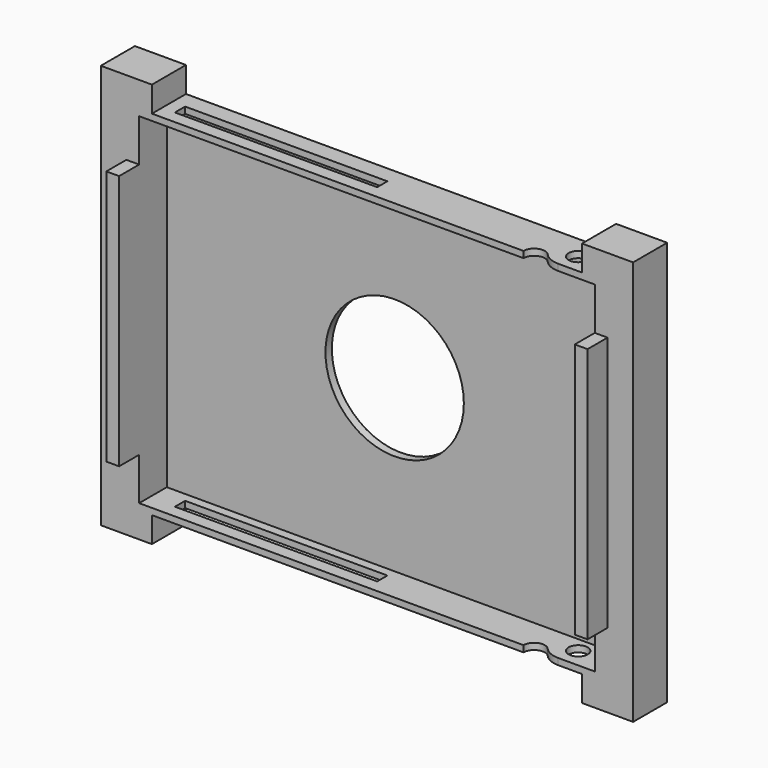
from build123d import *

# Parameters (mm, degrees)
F0_R      = 16.25
F1_DEPTH  = 15.875
F2_W      = 139.2096877098
F2_H      = 115.5483946204
F2_W_2    = 113
F2_H_2    = 80
F3_DEPTH  = 5.875
F4_W      = 107
F4_H      = 80
F5_DEPTH  = 14
F6_W      = 120.5911301091
F6_H      = 13.1527084535
F6_W_2    = 121.3300417974
F6_H_2    = 15.8128053223
F7_DEPTH  = 5.875
F8_R      = 1.5
F8_W      = 89
F8_H      = 3
F9_DEPTH  = 100
F10_W     = 42.4407012761
F10_H     = 10
F11_DEPTH = 1.5
F12_W     = 42.5221920013
F12_H     = 10
F13_DEPTH = 1.5
F14_R     = 2.5
F15_DEPTH = 95.5
F16_R     = 2.25
F17_DEPTH = 200
F18_R     = 5


with BuildPart() as f1:
    # F0 (on Front) → F1 (new body)
    with BuildSketch(Plane.XZ):
        Polygon((-50.5, 47.5), (-62.5, 47.5), (-62.5, -47.5), (-50.5, -47.5), (-50.5, -41.5), (50.5, -41.5), (50.5, -47.5), (62.5, -47.5), (62.5, 47.5), (50.5, 47.5), (50.5, 41.5), (-50.5, 41.5), align=None)
        Circle(F0_R, mode=Mode.SUBTRACT)
    extrude(amount=F1_DEPTH)

    # F2 (on face) → F3 (cut)
    with BuildSketch(Plane.XZ.offset(15.875)):
        Rectangle(F2_W, F2_H)
        Rectangle(F2_W_2, F2_H_2, mode=Mode.SUBTRACT)
    extrude(amount=-F3_DEPTH, mode=Mode.SUBTRACT)

    # F4 (on face) → F5 (cut)
    with BuildSketch(Plane.XZ.offset(15.875)):
        Rectangle(F4_W, F4_H)
    extrude(amount=-F5_DEPTH, mode=Mode.SUBTRACT)

    # F6 (on face) → F7 (cut)
    with BuildSketch(Plane.XZ.offset(15.875)):
        with Locations((0.0607829645, 36.5763542267)):
            Rectangle(F6_W, F6_H)
        with Locations((1.0213727103, -37.9064026611)):
            Rectangle(F6_W_2, F6_H_2)
    extrude(amount=-F7_DEPTH, mode=Mode.SUBTRACT)

    # F8 (on face) → F9 (cut)
    with BuildSketch(Plane.XY.offset(41.5)):
        with Locations((46, -5.5)):
            Circle(F8_R)
        with Locations((-3, -5.5)):
            Rectangle(F8_W, F8_H)
    extrude(amount=-F9_DEPTH, mode=Mode.SUBTRACT)

    # F10 (on face) → F11 (join)
    with BuildSketch(Plane.XY.offset(41.5)):
        with Locations((21.220350638, -5)):
            Rectangle(F10_W, F10_H)
    extrude(amount=-F11_DEPTH)

    # F12 (on face) → F13 (join)
    with BuildSketch(Plane(origin=(0, 0, -41.5), x_dir=(1, 0, 0), z_dir=(0, 0, -1))):
        with Locations((21.2610960007, 5)):
            Rectangle(F12_W, F12_H)
    extrude(amount=-F13_DEPTH)

    # F14 (on face) → F15 (cut)
    with BuildSketch(Plane(origin=(0, 0, -41.5), x_dir=(1, 0, 0), z_dir=(0, 0, -1))):
        with Locations((39.25, 10)):
            Circle(F14_R)
    extrude(amount=-F15_DEPTH, mode=Mode.SUBTRACT)

    # F16 (on face) → F17 (cut)
    with BuildSketch(Plane.XY.offset(41.5)):
        with Locations((46, -5.5)):
            Circle(F16_R)
    extrude(amount=-F17_DEPTH, mode=Mode.SUBTRACT)

    # F18
    f18_edges = [f1.edges().sort_by_distance(p)[0] for p in [
        (41.75, -10, -40.75),
        (41.75, -10, 40.75),
    ]]
    fillet(f18_edges, radius=F18_R)


solid = f1.part
